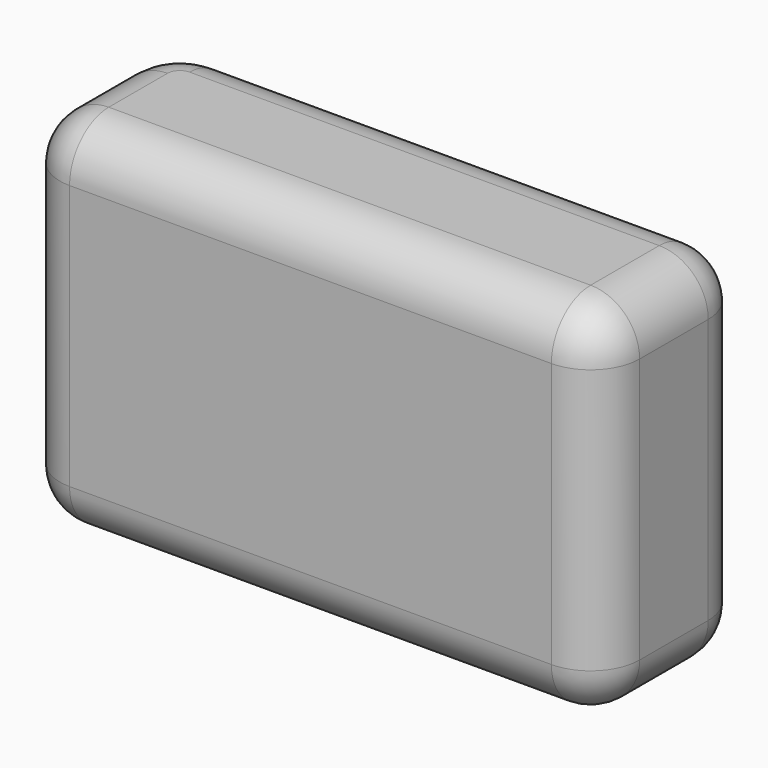
from build123d import *

# Parameters (mm, degrees)
F0_W        = 47.3195426166
F0_H        = 29.6245701611
F1_DEPTH    = 15
F2_R        = 4
F3_T1_DEPTH = 29.6245701611
F3_T4_ANGLE = 90
F3_T6_ANGLE = 90


# Not quite as in the source:
# - a fillet or chamfer that OpenCascade refuses, or shapes differently, is made with other operations: its cross-section is extruded or revolved along the edge and cut away or added


with BuildPart() as f1:
    # F0 (on Front) → F1 (new body)
    with BuildSketch(Plane.XZ):
        with Locations((-42.1840865165, -1.9065886736)):
            Rectangle(F0_W, F0_H)
    extrude(amount=F1_DEPTH)

    # F2
    f2_edges = [f1.edges().sort_by_distance(p)[0] for p in [
        (-42.184087, -15, 12.905696),
        (-65.843858, -15, -1.906589),
        (-42.184087, -15, -16.718874),
        (-18.524315, -15, -1.906589),
        (-18.524315, -7.5, 12.905696),
        (-42.184087, 0, 12.905696),
        (-18.524315, -7.5, -16.718874),
        (-18.524315, 0, -1.906589),
        (-42.184087, 0, -16.718874),
        (-65.843858, -7.5, -16.718874),
        (-65.843858, -7.5, 12.905696),
    ]]
    fillet(f2_edges, radius=F2_R)

    # F3: fillet of radius 5 on 1 edges, made by hand

    # F3_s2 → F3_t1 (cut)
    with BuildSketch(Plane.XY.offset(-16.7188737541)):
        with BuildLine():
            ThreePointArc((-65.8438578248, -5), (-64.3793917307, -1.4644660941), (-60.8438578248, 0))
            Line((-60.8438578248, 0), (-65.8438578248, 0))
            Line((-65.8438578248, 0), (-65.8438578248, -5))
        make_face()
    extrude(amount=F3_T1_DEPTH, mode=Mode.SUBTRACT)

    # F3_s3 → F3_t4 (revolve, cut)
    with BuildSketch(Plane.YZ.offset(-60.8438578248)):
        with BuildLine():
            ThreePointArc((-4, 12.905696407), (-1.1715728753, 11.7341235317), (0, 8.905696407))
            Line((0, 8.905696407), (0, 12.905696407))
            Line((0, 12.905696407), (-4, 12.905696407))
        make_face()
    revolve(axis=Axis((-60.8438578248, -5, 12.905696407), (0, 0, 1)), revolution_arc=F3_T4_ANGLE, mode=Mode.SUBTRACT)

    # F3_s5 → F3_t6 (revolve, cut)
    with BuildSketch(Plane.XZ.offset(5)):
        with BuildLine():
            ThreePointArc((-61.8438578248, -16.7188737541), (-64.6722849495, -15.5473008789), (-65.8438578248, -12.7188737541))
            Line((-65.8438578248, -12.7188737541), (-65.8438578248, -16.7188737541))
            Line((-65.8438578248, -16.7188737541), (-61.8438578248, -16.7188737541))
        make_face()
    revolve(axis=Axis((-60.8438578248, -5, -16.7188737541), (0, 0, -1)), revolution_arc=F3_T6_ANGLE, mode=Mode.SUBTRACT)


solid = f1.part
